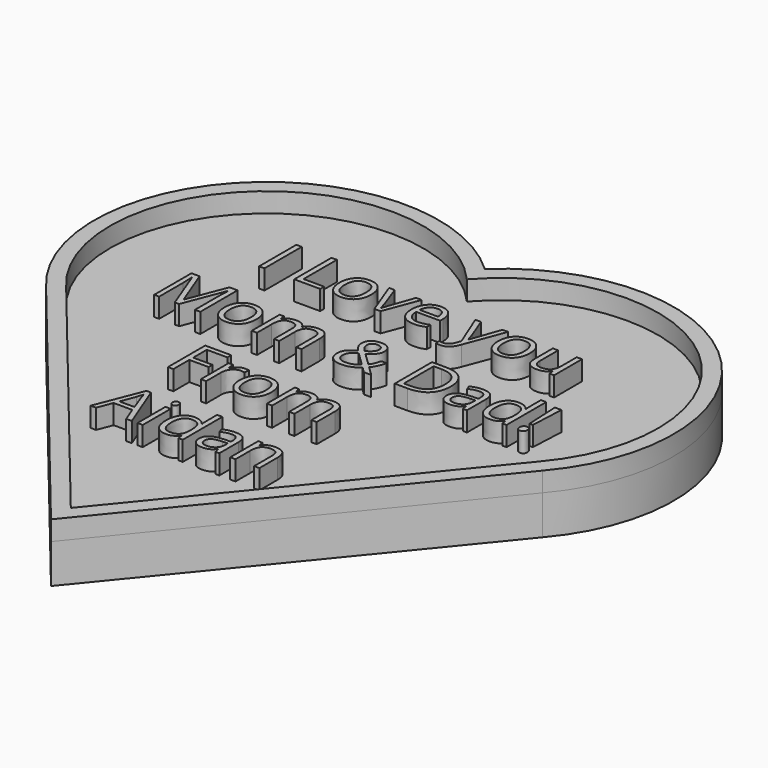
from build123d import *

# Parameters (mm, degrees)
F2_DEPTH     = 6.35
F3_DEPTH     = 3.175
F1_TEXT_SIZE = 10.5833333333
F4_DEPTH     = 3.175


# Not quite as in the source:
# - Text() gives the source's letters only with a copy of the font that has no kerning and outlines rounded to 1/6400 em; it was checked with that copy


with BuildPart() as f2:
    # F0 (on Top) → F2 (new body)
    with BuildSketch(Plane.XY):
        with BuildLine():
            ThreePointArc((40.2598806708, -18.1874837662), (38.3932700049, 20.1613865925), (0, 20.4387158064))
            ThreePointArc((0, 20.4387158064), (-38.3932700049, 20.1613865925), (-40.2598806708, -18.1874837662))
            Line((-40.2598806708, -18.1874837662), (0, -67.5171474962))
            Line((0, -67.5171474962), (40.2598806708, -18.1874837662))
        make_face()
        with BuildLine():
            ThreePointArc((-38.3120624414, -16.556960787), (-35.7290778372, 19.1564183109), (0, 16.8005208253))
            ThreePointArc((0, 16.8005208253), (35.7290778372, 19.1564183109), (38.3120624414, -16.556960787))
            Line((38.3120624414, -16.556960787), (0, -63.5))
            Line((0, -63.5), (-38.3120624414, -16.556960787))
        make_face(mode=Mode.SUBTRACT)
        with BuildLine():
            ThreePointArc((38.3120624414, -16.556960787), (35.7290778372, 19.1564183109), (0, 16.8005208253))
            ThreePointArc((0, 16.8005208253), (-35.7290778372, 19.1564183109), (-38.3120624414, -16.556960787))
            Line((-38.3120624414, -16.556960787), (0, -63.5))
            Line((0, -63.5), (38.3120624414, -16.556960787))
        make_face()
    extrude(amount=-F2_DEPTH)

    # F1 (on Top) → F4 (join)
    with BuildSketch(Plane.XY):
        with Locations((-23.814857123, 3.1405028379)):
            Text('I Love you', F1_TEXT_SIZE, font='Open Sans', text_align=(TextAlign.LEFT, TextAlign.BOTTOM))
        with Locations((-29.3148831647, -11.2528304954)):
            Text('Mom & Dad!', F1_TEXT_SIZE, font='Open Sans', text_align=(TextAlign.LEFT, TextAlign.BOTTOM))
        with Locations((-15.5648180605, -25.6461638287)):
            Text('From', F1_TEXT_SIZE, font='Open Sans', text_align=(TextAlign.LEFT, TextAlign.BOTTOM))
        with Locations((-15.5648180605, -40.0394971621)):
            Text('Aidan', F1_TEXT_SIZE, font='Open Sans', text_align=(TextAlign.LEFT, TextAlign.BOTTOM))
    extrude(amount=F4_DEPTH)


with BuildPart() as f3:
    # F0 (on Top) → F3 (new body)
    with BuildSketch(Plane.XY):
        with BuildLine():
            ThreePointArc((40.2598806708, -18.1874837662), (38.3932700049, 20.1613865925), (0, 20.4387158064))
            ThreePointArc((0, 20.4387158064), (-38.3932700049, 20.1613865925), (-40.2598806708, -18.1874837662))
            Line((-40.2598806708, -18.1874837662), (0, -67.5171474962))
            Line((0, -67.5171474962), (40.2598806708, -18.1874837662))
        make_face()
        with BuildLine():
            ThreePointArc((-38.3120624414, -16.556960787), (-35.7290778372, 19.1564183109), (0, 16.8005208253))
            ThreePointArc((0, 16.8005208253), (35.7290778372, 19.1564183109), (38.3120624414, -16.556960787))
            Line((38.3120624414, -16.556960787), (0, -63.5))
            Line((0, -63.5), (-38.3120624414, -16.556960787))
        make_face(mode=Mode.SUBTRACT)
    extrude(amount=F3_DEPTH)


solid = Compound([f2.part, f3.part])
